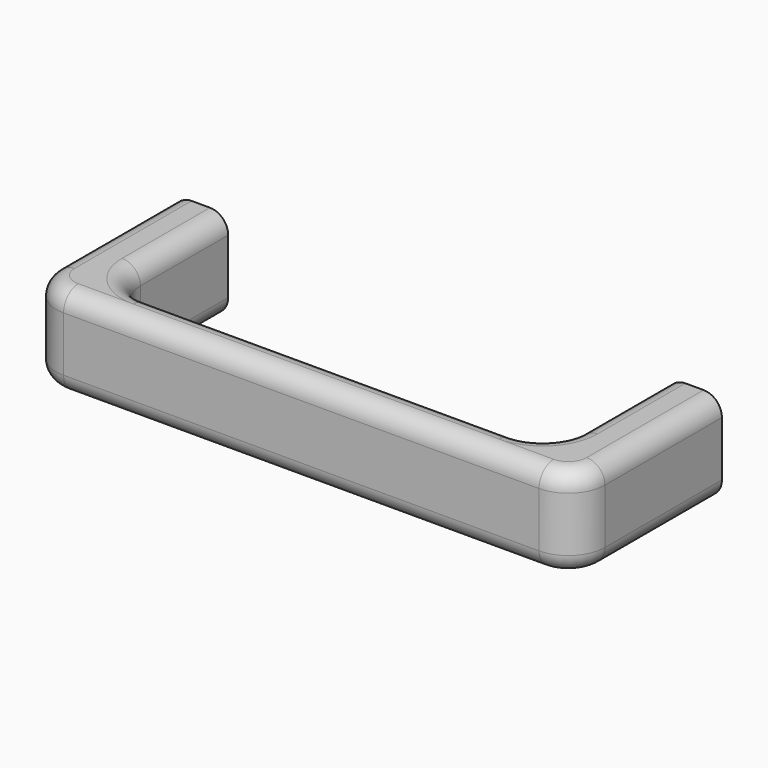
from build123d import *

# Parameters (mm, degrees)
F1_DEPTH = 25
F2_R     = 4.99999
F4_D     = 8
F4_DEPTH = 12
F4_TIP   = 2.4034424761
F6_D     = 8
F6_DEPTH = 12
F6_TIP   = 2.4034424761


# Not quite as in the source:
# - a fillet or chamfer is up to 0.001 mm smaller than in the source, because OpenCascade refuses the exact size


with BuildPart() as f1:
    # F0 (on Top) → F1 (new body)
    with BuildSketch(Plane.XY):
        with BuildLine():
            Line((75, -15), (75, 25))
            Line((75, 25), (60, 25))
            Line((60, 25), (60, -5))
            ThreePointArc((60, -5), (57.0710678119, -12.0710678119), (50, -15))
            Line((50, -15), (-50, -15))
            ThreePointArc((-50, -15), (-57.0710678119, -12.0710678119), (-60, -5))
            Line((-60, -5), (-60, 25))
            Line((-60, 25), (-75, 25))
            Line((-75, 25), (-75, -15))
            ThreePointArc((-75, -15), (-72.0710678119, -22.0710678119), (-65, -25))
            Line((-65, -25), (65, -25))
            ThreePointArc((65, -25), (72.0710678119, -22.0710678119), (75, -15))
        make_face()
    extrude(amount=F1_DEPTH)

    # F2 (radius 5 in the source; OpenCascade refuses exactly that, so slightly less here)
    f2_edges = [f1.edges().sort_by_distance(p)[0] for p in [
        (-57.071068, -12.071068, 0),
        (-57.071068, -12.071068, 25),
        (-72.071068, -22.071068, 0),
        (-72.071068, -22.071068, 25),
    ]]
    fillet(f2_edges, radius=F2_R)

    # F4
    with Locations(Plane(origin=(0, 25, 0), x_dir=(-1, 0, 0), z_dir=(0, 1, 0))):
        with Locations((67.5, 12.5)):
            Hole(F4_D / 2, depth=F4_DEPTH)
            with Locations((0, 0, -(F4_DEPTH + F4_TIP / 2))):  # 118° drill point
                Cone(0, F4_D / 2, F4_TIP, mode=Mode.SUBTRACT)

    # F6
    with Locations(Plane(origin=(0, 25, 0), x_dir=(-1, 0, 0), z_dir=(0, 1, 0))):
        with Locations((-67.5, 12.5)):
            Hole(F6_D / 2, depth=F6_DEPTH)
            with Locations((0, 0, -(F6_DEPTH + F6_TIP / 2))):  # 118° drill point
                Cone(0, F6_D / 2, F6_TIP, mode=Mode.SUBTRACT)


solid = f1.part
